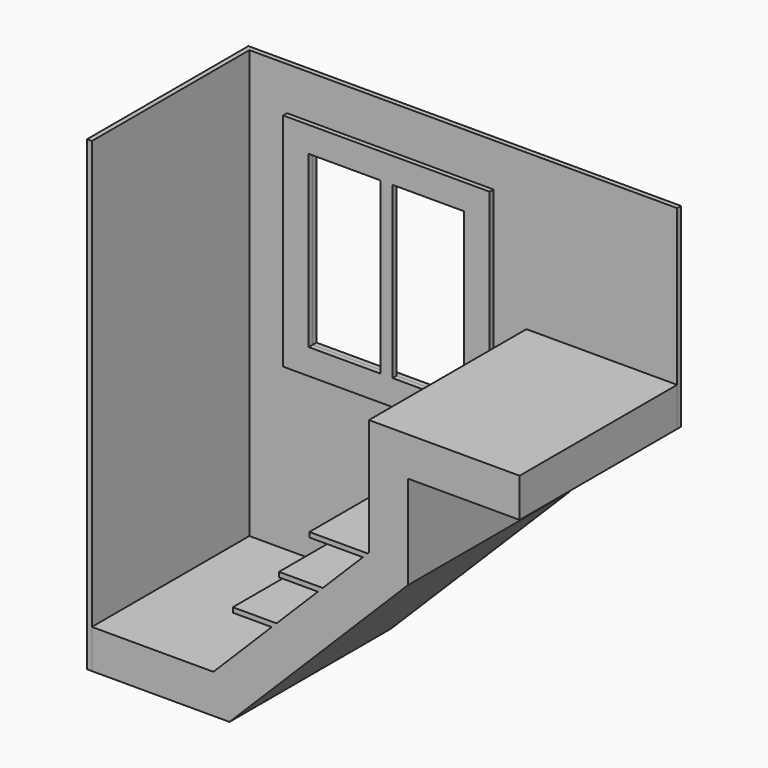
from build123d import *

# Parameters (mm, degrees)
F1_DEPTH = 514.35
F2_W     = 1028.7
F2_H     = 203.2
F2_H_2   = 2235.2
F3_DEPTH = 25.4
F5_DEPTH = 25.4
F6_W     = 812.8
F6_H     = 889
F7_DEPTH = 25.401
F8_W     = 1079.5
F8_H     = 1155.7
F8_W_2   = 63.5
F8_H_2   = 889
F9_DEPTH = 25.4


with BuildPart() as f1:
    # F0 (on Front) → F1 (new body, symmetric)
    with BuildSketch(Plane.XZ):
        Polygon((2235.2, 1422.4), (2235.2, 1625.6), (1447.8, 1625.6), (1447.8, 1016), (1441.45, 1009.65), (1136.65, 1009.65), (1136.65, 984.25), (1416.05, 984.25), (1206.5, 774.7), (977.9, 774.7), (977.9, 749.3), (1181.1, 749.3), (965.2, 533.4), (736.6, 533.4), (736.6, 508), (939.8, 508), (635, 203.2), (0, 203.2), (0, 0), (719.1681958742, 0), (1651, 931.8318041258), (1651, 1422.4), align=None)
    extrude(amount=F1_DEPTH, both=True)


with BuildPart() as f3:
    # F2 (on face) → F3 (new body)
    with BuildSketch(Plane(origin=(0, 0, 0), x_dir=(0, -1, 0), z_dir=(-1, 0, 0))):
        with Locations((0, 101.6)):
            Rectangle(F2_W, F2_H)
        with Locations((0, 1320.8)):
            Rectangle(F2_W, F2_H_2)
    extrude(amount=F3_DEPTH)

    # F4 (on face) → F5 (join)
    with BuildSketch(Plane(origin=(0, 514.35, 0), x_dir=(-1, 0, 0), z_dir=(0, 1, 0))):
        Polygon((-2235.2, 2438.4), (-2235.2, 1625.6), (-1447.8, 1625.6), (-1447.8, 1016), (-1441.45, 1009.65), (-1136.65, 1009.65), (-1136.65, 984.25), (-1416.05, 984.25), (-1206.5, 774.7), (-977.9, 774.7), (-977.9, 749.3), (-1181.1, 749.3), (-965.2, 533.4), (-736.6, 533.4), (-736.6, 508), (-939.8, 508), (-635, 203.2), (0, 203.2), (0, 0), (25.4, 0), (25.4, 2438.4), align=None)
        Polygon((-2235.2, 1625.6), (-2235.2, 1422.4), (-1651, 1422.4), (-1651, 931.8318041258), (-719.1681958742, 0), (0, 0), (0, 203.2), (-635, 203.2), (-939.8, 508), (-736.6, 508), (-736.6, 533.4), (-965.2, 533.4), (-1181.1, 749.3), (-977.9, 749.3), (-977.9, 774.7), (-1206.5, 774.7), (-1416.05, 984.25), (-1136.65, 984.25), (-1136.65, 1009.65), (-1441.45, 1009.65), (-1447.8, 1016), (-1447.8, 1625.6), align=None)
    extrude(amount=F5_DEPTH)

    # F6 (on face) → F7 (cut, through all)
    with BuildSketch(Plane.XZ.offset(-514.35)):
        with Locations((736.6, 1634.46784906)):
            Rectangle(F6_W, F6_H)
    extrude(amount=-F7_DEPTH, mode=Mode.SUBTRACT)


with BuildPart() as f9:
    # F8 (on face) → F9 (new body)
    with BuildSketch(Plane.XZ.offset(-514.35)):
        with Locations((736.6, 1634.46784906)):
            Rectangle(F8_W, F8_H)
        Polygon((704.85, 1189.96784906), (330.2, 1189.96784906), (330.2, 2078.96784906), (704.85, 2078.96784906), (768.35, 2078.96784906), (1143, 2078.96784906), (1143, 1189.96784906), (768.35, 1189.96784906), align=None, mode=Mode.SUBTRACT)
        with Locations((736.6, 1634.46784906)):
            Rectangle(F8_W_2, F8_H_2)
    extrude(amount=F9_DEPTH)


solid = Compound([f1.part, f3.part, f9.part])
